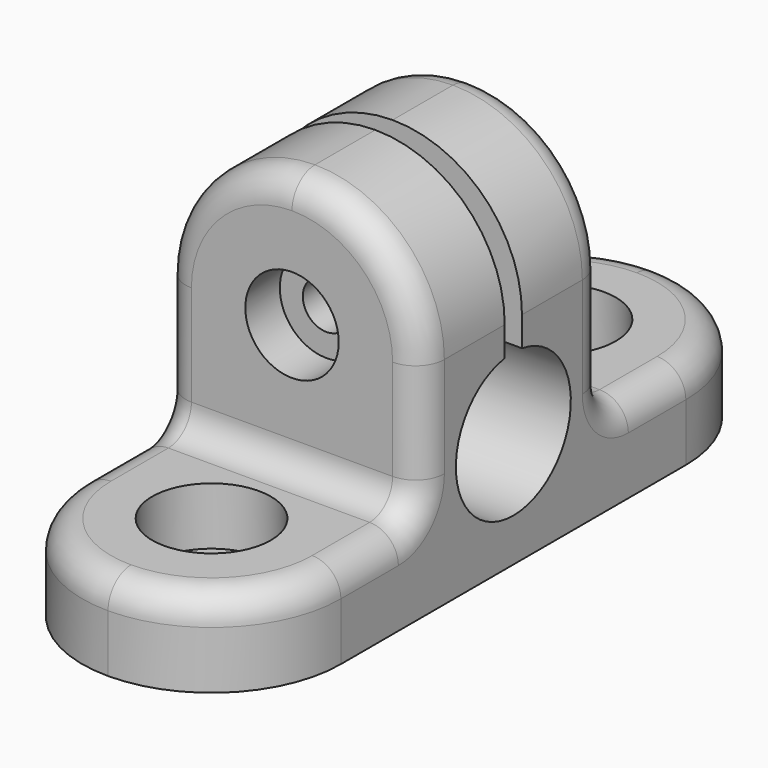
from build123d import *

# Parameters (mm, degrees)
F1_DEPTH       = 18
F4_D           = 4.4
F4_CBORE_D     = 8.25
F4_CBORE_DEPTH = 4
F5_R           = 8.99999
F6_R           = 2
F7_D           = 3.3
F7_CBORE_D     = 6.5
F7_CBORE_DEPTH = 3
F9_DEPTH       = 3


# Not quite as in the source:
# - a fillet or chamfer is up to 0.001 mm smaller than in the source, because OpenCascade refuses the exact size


with BuildPart() as f1:
    # F0 (on Right) → F1 (new body)
    with BuildSketch(Plane.YZ):
        with BuildLine():
            Line((0, 6), (0, 0))
            Line((0, 0), (48, 0))
            Line((48, 0), (48, 6))
            Line((48, 6), (34, 6))
            ThreePointArc((34, 6), (32.5857864376, 6.5857864376), (32, 8))
            Line((32, 8), (32, 24))
            Line((32, 24), (24.75, 24))
            Line((24.75, 24), (24.75, 12.9434299833))
            ThreePointArc((24.75, 12.9434299833), (24, 3), (23.25, 12.9434299833))
            Line((23.25, 12.9434299833), (23.25, 24))
            Line((23.25, 24), (16, 24))
            Line((16, 24), (16, 8))
            ThreePointArc((16, 8), (15.4142135624, 6.5857864376), (14, 6))
            Line((14, 6), (0, 6))
        make_face()
    extrude(amount=F1_DEPTH)

    # F4 (through all)
    with Locations(Plane.XY.offset(6)):
        with Locations((9, 9), (9, 39)):
            CounterBoreHole(F4_D / 2, F4_CBORE_D / 2, F4_CBORE_DEPTH)

    # F5 (radius 9 in the source; OpenCascade refuses exactly that, so slightly less here)
    f5_edges = [f1.edges().sort_by_distance(p)[0] for p in [
        (18, 0, 3),
        (0, 0, 3),
        (18, 48, 3),
        (0, 48, 3),
        (0, 28.375, 24),
        (0, 19.625, 24),
        (18, 19.625, 24),
        (18, 28.375, 24),
    ]]
    fillet(f5_edges, radius=F5_R)

    # F6
    f6_edges = [f1.edges().sort_by_distance(p)[0] for p in [
        (18, 11.499995, 6),
        (18, 36.500005, 6),
    ]]
    fillet(f6_edges, radius=F6_R)

    # F7 (through all)
    with Locations(Plane.XZ.offset(-16)):
        with Locations((9, 15)):
            CounterBoreHole(F7_D / 2, F7_CBORE_D / 2, F7_CBORE_DEPTH)

    # F8 (on face) → F9 (cut)
    with BuildSketch(Plane(origin=(0, 32, 0), x_dir=(-1, 0, 0), z_dir=(0, 1, 0))):
        Polygon((-6, 13.2679491924), (-6, 16.7320508076), (-9, 18.4641016151), (-12, 16.7320508076), (-12, 13.2679491924), (-9, 11.5358983849), align=None)
    extrude(amount=-F9_DEPTH, mode=Mode.SUBTRACT)


solid = f1.part
